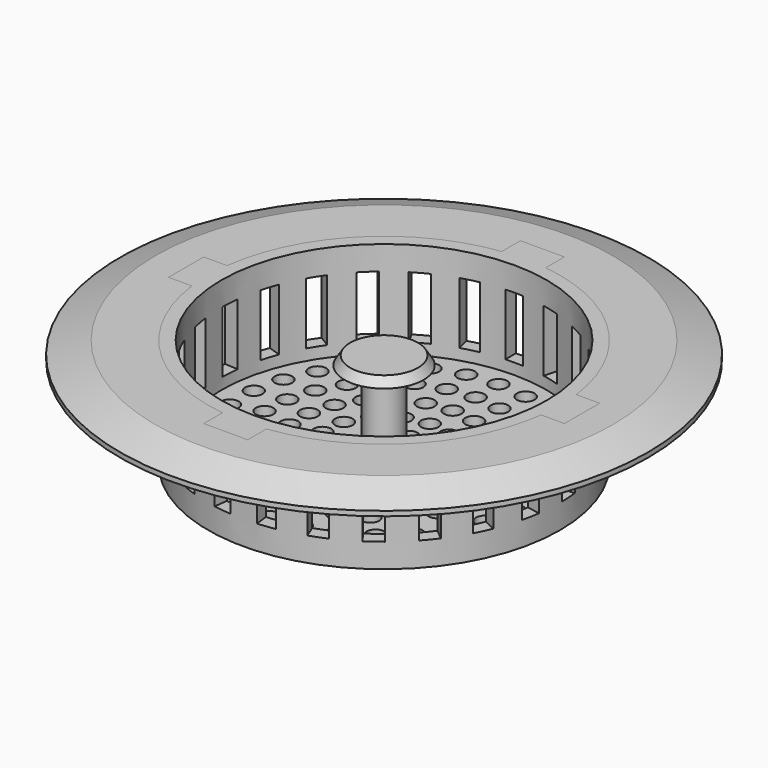
from build123d import *

# Parameters (mm, degrees)
F0_R      = 40
F1_DEPTH  = 25
F2_T      = -3
F4_DEPTH  = 2
F5_R      = 60
F5_R_2    = 40
F6_DEPTH  = 4
F7_DEPTH  = 2
F8_R      = 2
F9_DEPTH  = 3.001
F12_SIZE2 = 2.9117618741
F12_SIZE  = 8
F14_W     = 4
F14_H     = 6.67
F15_DEPTH = 7


# Not quite as in the source:
# - a feature names something its author has since deleted; it is built from what else it names


with BuildPart() as f1:
    # F0 (on Top) → F1 (new body)
    with BuildSketch(Plane.XY):
        Circle(F0_R)
    extrude(amount=F1_DEPTH)

    # F2
    f2_openings = [f1.faces().sort_by_distance(p)[0] for p in [
        (0, 0, 25),
    ]]
    offset(amount=F2_T, openings=f2_openings)

    # F3 (on face) → F4 (join)
    with BuildSketch(Plane.XY.offset(25)):
        with BuildLine():
            ThreePointArc((-39.686269666, -5), (-40, 0), (-39.686269666, 5))
            Line((-39.686269666, 5), (-45, 5))
            Line((-45, 5), (-45, 0))
            Line((-45, 0), (-45, -5))
            Line((-45, -5), (-39.686269666, -5))
        make_face()
        with BuildLine():
            Line((-5, 45), (-5, 39.686269666))
            ThreePointArc((-5, 39.686269666), (0, 40), (5, 39.686269666))
            Line((5, 39.686269666), (5, 45))
            Line((5, 45), (0, 45))
            Line((0, 45), (-5, 45))
        make_face()
        with BuildLine():
            Line((45, 5), (39.686269666, 5))
            ThreePointArc((39.686269666, 5), (39.9214903695, 2.5049165017), (40, 0))
            ThreePointArc((40, 0), (39.9214903695, -2.5049165017), (39.686269666, -5))
            Line((39.686269666, -5), (45, -5))
            Line((45, -5), (45, 0))
            Line((45, 0), (45, 5))
        make_face()
        with BuildLine():
            ThreePointArc((5, -39.686269666), (0, -40), (-5, -39.686269666))
            Line((-5, -39.686269666), (-5, -45))
            Line((-5, -45), (0, -45))
            Line((0, -45), (5, -45))
            Line((5, -45), (5, -39.686269666))
        make_face()
    extrude(amount=-F4_DEPTH)

    # F8 (on face) → F9 (cut, through all)
    with BuildSketch(Plane.XY.offset(3)):
        with Locations((30.9093367796, -10.0430523172)):
            Circle(F8_R)
        with Locations((-19.1030206995, 26.2930523172)):
            Circle(F8_R)
        with Locations((-14.2872334298, -21.7226830967)):
            Circle(F8_R)
        with Locations((-24.9077273202, -7.4568840505)):
            Circle(F8_R)
        with Locations((32.3219615995, -3.3971750562)):
            Circle(F8_R)
        with Locations((-5.4728203773, 4.364428613)):
            Circle(F8_R)
        with Locations((0, 7)):
            Circle(F8_R)
        with Locations((28.145825623, -16.25)):
            Circle(F8_R)
        with Locations((-5.9960126393, 25.2991666351)):
            Circle(F8_R)
        with Locations((32.3219615995, 3.3971750562)):
            Circle(F8_R)
        with Locations((-2.7028519806, -12.7159188095)):
            Circle(F8_R)
        with Locations((16.7124778519, 19.9171555211)):
            Circle(F8_R)
        with Locations((10.5424959404, 16.4044438902)):
            Circle(F8_R)
        with Locations((14.7371166999, 12.7697843119)):
            Circle(F8_R)
        with Locations((30.9093367796, 10.0430523172)):
            Circle(F8_R)
        with Locations((-6.7571299516, -31.7897970238)):
            Circle(F8_R)
        with Locations((-13.2189409, 29.6902273734)):
            Circle(F8_R)
        with Locations((-11.6687786852, 23.2344486484)):
            Circle(F8_R)
        with Locations((19.3015181167, -2.7751393463)):
            Circle(F8_R)
        with Locations((11.6687786852, 23.2344486484)):
            Circle(F8_R)
        with Locations((23.8736187789, 10.298073917)):
            Circle(F8_R)
        with Locations((-23.8736187789, 10.298073917)):
            Circle(F8_R)
        with Locations((-12.3637347118, 4.0172209269)):
            Circle(F8_R)
        with Locations((-30.9093367796, 10.0430523172)):
            Circle(F8_R)
        with Locations((-5.28757636, 11.8760909494)):
            Circle(F8_R)
        with Locations((-11.2583302492, -6.5)):
            Circle(F8_R)
        with Locations((-16.7124778519, 19.9171555211)):
            Circle(F8_R)
        with Locations((-30.9093367796, -10.0430523172)):
            Circle(F8_R)
        with Locations((0, -32.5)):
            Circle(F8_R)
        with Locations((-22.5166604984, -13)):
            Circle(F8_R)
        with Locations((-28.145825623, 16.25)):
            Circle(F8_R)
        with Locations((-14.7371166999, 12.7697843119)):
            Circle(F8_R)
        with Locations((0, 19.5)):
            Circle(F8_R)
        with Locations((0, 26)):
            Circle(F8_R)
        with Locations((7.6412082798, -10.5172209269)):
            Circle(F8_R)
        with Locations((-8.8925237265, -24.4320081404)):
            Circle(F8_R)
        with Locations((-32.3219615995, 3.3971750562)):
            Circle(F8_R)
        with Locations((-19.1030206995, -26.2930523172)):
            Circle(F8_R)
        with Locations((12.3637347118, 4.0172209269)):
            Circle(F8_R)
        with Locations((-3.0184157673, -25.8241973013)):
            Circle(F8_R)
        with Locations((3.0371861738, -6.3067820753)):
            Circle(F8_R)
        with Locations((14.2872334298, -21.7226830967)):
            Circle(F8_R)
        with Locations((-20.8552030116, 15.5261233843)):
            Circle(F8_R)
        with Locations((-25.9560121151, -1.5117655517)):
            Circle(F8_R)
        with Locations((-19.3015181167, -2.7751393463)):
            Circle(F8_R)
        with Locations((24.152206828, -21.7467447067)):
            Circle(F8_R)
        with Locations((8.8925237265, -24.4320081404)):
            Circle(F8_R)
        with Locations((11.2583302492, -6.5)):
            Circle(F8_R)
        with Locations((-6.7571299516, 31.7897970238)):
            Circle(F8_R)
        with Locations((6.7571299516, 31.7897970238)):
            Circle(F8_R)
        with Locations((12.9287846398, -1.3588700225)):
            Circle(F8_R)
        with Locations((5.4937848584, 18.7101129855)):
            Circle(F8_R)
        with Locations((3.0184157673, -25.8241973013)):
            Circle(F8_R)
        with Locations((25.9560121151, -1.5117655517)):
            Circle(F8_R)
        with Locations((-18.9117146809, -17.8422825846)):
            Circle(F8_R)
        with Locations((28.145825623, 16.25)):
            Circle(F8_R)
        with Locations((-7.6412082798, -10.5172209269)):
            Circle(F8_R)
        with Locations((-6.8244953853, -1.5576465377)):
            Circle(F8_R)
        with Locations((25.6050015783, 4.5148526193)):
            Circle(F8_R)
        with Locations((0, 32.5)):
            Circle(F8_R)
        with Locations((-32.3219615995, -3.3971750562)):
            Circle(F8_R)
        with Locations((-10.5424959404, 16.4044438902)):
            Circle(F8_R)
        with Locations((24.152206828, 21.7467447067)):
            Circle(F8_R)
        with Locations((-25.6050015783, 4.5148526193)):
            Circle(F8_R)
        with Locations((5.28757636, 11.8760909494)):
            Circle(F8_R)
        with Locations((13.2189409, 29.6902273734)):
            Circle(F8_R)
        with Locations((19.1030206995, 26.2930523172)):
            Circle(F8_R)
        with Locations((-9.6608827312, 8.6986978827)):
            Circle(F8_R)
        with Locations((-19.3015181167, 2.7751393463)):
            Circle(F8_R)
        with Locations((-10.5424959404, -16.4044438902)):
            Circle(F8_R)
        with Locations((-24.152206828, -21.7467447067)):
            Circle(F8_R)
        with Locations((5.4728203773, 4.364428613)):
            Circle(F8_R)
        with Locations((9.6608827312, 8.6986978827)):
            Circle(F8_R)
        with Locations((0, 13)):
            Circle(F8_R)
        with Locations((19.1030206995, -26.2930523172)):
            Circle(F8_R)
        with Locations((13.2189409, -29.6902273734)):
            Circle(F8_R)
        with Locations((6.7571299516, -31.7897970238)):
            Circle(F8_R)
        with Locations((22.5166604984, -13)):
            Circle(F8_R)
        with Locations((24.9077273202, -7.4568840505)):
            Circle(F8_R)
        with Locations((18.9117146809, -17.8422825846)):
            Circle(F8_R)
        with Locations((-17.7378239094, -8.1005927535)):
            Circle(F8_R)
        with Locations((-17.7378239094, 8.1005927535)):
            Circle(F8_R)
        with Locations((-14.7371166999, -12.7697843119)):
            Circle(F8_R)
        with Locations((10.5424959404, -16.4044438902)):
            Circle(F8_R)
        with Locations((14.7371166999, -12.7697843119)):
            Circle(F8_R)
        with Locations((17.7378239094, 8.1005927535)):
            Circle(F8_R)
        with Locations((20.8552030116, 15.5261233843)):
            Circle(F8_R)
        with Locations((5.9960126393, 25.2991666351)):
            Circle(F8_R)
        with Locations((-5.4937848584, 18.7101129855)):
            Circle(F8_R)
        with Locations((-28.145825623, -16.25)):
            Circle(F8_R)
        with Locations((-24.152206828, 21.7467447067)):
            Circle(F8_R)
        with Locations((0, -19.5)):
            Circle(F8_R)
        with Locations((5.4937848584, -18.7101129855)):
            Circle(F8_R)
        with Locations((-12.9287846398, -1.3588700225)):
            Circle(F8_R)
        with Locations((6.8244953853, -1.5576465377)):
            Circle(F8_R)
        with Locations((-13.2189409, -29.6902273734)):
            Circle(F8_R)
        with Locations((17.7378239094, -8.1005927535)):
            Circle(F8_R)
        with Locations((2.7028519806, -12.7159188095)):
            Circle(F8_R)
        with Locations((-5.4937848584, -18.7101129855)):
            Circle(F8_R)
        with Locations((19.3015181167, 2.7751393463)):
            Circle(F8_R)
        with Locations((-3.0371861738, -6.3067820753)):
            Circle(F8_R)
    extrude(amount=-F9_DEPTH, mode=Mode.SUBTRACT)

    # F10 (on Front) → F11 (revolve)
    with BuildSketch(Plane.XZ):
        Polygon((0, 22), (0, 0), (4, 0), (4, 20), (9, 20), (7.7110708915, 22), align=None)
    revolve(axis=Axis((0, 0, 12.5114747789), (0, 0, -1)))

    # F14 (on offset) → F15 (cut, symmetric)
    with BuildSketch(Plane.XY.offset(12.5)):
        Polygon((-6.4256858452, -34.9070814551), (-7.2616585131, -41.5244865129), (-3.2931997078, -42.0258194471), (-2.45722704, -35.4084143894), align=None)
        with Locations((0, 38.7721806765)):
            Rectangle(F14_W, F14_H)
        Polygon((-15.3193786306, 32.0173454969), (-18.5326756369, 37.8623110528), (-22.037902357, 35.9352963564), (-18.8246053508, 30.0903308005), align=None)
        Polygon((11.1857433132, -33.6849064245), (13.6411340796, -39.8865155854), (17.3602400231, -38.4140173747), (14.9048492567, -32.2124082138), align=None)
        Polygon((-22.8004822195, 27.2016871693), (-27.366411416, 32.0639079142), (-30.2822859257, 29.3257194904), (-25.7163567292, 24.4634987455), align=None)
        Polygon((19.2114181957, -29.8448519046), (23.1319458285, -35.2409952571), (26.368013806, -32.8898542479), (22.4474861732, -27.4937108954), align=None)
        Polygon((26.0299690184, -24.1295355778), (31.1692923477, -28.3811535894), (33.7189883067, -25.2991006183), (28.5796649773, -21.0474826067), align=None)
        Polygon((18.8246053508, 30.0903308005), (22.037902357, 35.9352963564), (18.5326756369, 37.8623110528), (15.3193786306, 32.0173454969), align=None)
        Polygon((2.45722704, -35.4084143894), (3.2931997078, -42.0258194471), (7.2616585131, -41.5244865129), (6.4256858452, -34.9070814551), align=None)
        Polygon((30.9922548362, 17.299535094), (36.6239220993, 20.8734998165), (34.4806149193, 24.2508115185), (28.8489476562, 20.676846796), align=None)
        Polygon((-28.8489476562, 20.676846796), (-34.4806149193, 24.2508115185), (-36.6239220993, 20.8734998165), (-30.9922548362, 17.299535094), align=None)
        Polygon((-35.2416724562, 4.2211724422), (-41.8985107348, 4.6399852074), (-42.1496728129, 0.6478782937), (-35.4928345343, 0.2290655285), align=None)
        Polygon((10.7500347861, 33.8264767068), (12.4087963335, 40.2869263915), (8.534463689, 41.2816859402), (6.8757021416, 34.8212362554), align=None)
        Polygon((-22.4474861732, -27.4937108954), (-26.368013806, -32.8898542479), (-23.1319458285, -35.2409952571), (-19.2114181957, -29.8448519046), align=None)
        Polygon((-14.9048492567, -32.2124082138), (-17.3602400231, -38.4140173747), (-13.6411340796, -39.8865155854), (-11.1857433132, -33.6849064245), align=None)
        Polygon((-6.8757021416, 34.8212362554), (-8.534463689, 41.2816859401), (-12.4087963335, 40.2869263915), (-10.7500347861, 33.8264767068), align=None)
        Polygon((-33.0847276127, 12.8528040944), (-39.4282745764, 14.9139474468), (-40.6643425539, 11.1097213817), (-34.3207955902, 9.0485780292), align=None)
        Polygon((25.7163567292, 24.4634987455), (30.2822859257, 29.3257194904), (27.366411416, 32.0639079142), (22.8004822195, 27.2016871693), align=None)
        Polygon((35.4928345343, 0.2290655285), (42.1496728129, 0.6478782937), (41.8985107348, 4.6399852074), (35.2416724562, 4.2211724422), align=None)
        Polygon((-32.9160783223, -13.2787635786), (-38.9512747623, -16.1187114533), (-37.248157596, -19.7380196632), (-31.2129611561, -16.8980717884), align=None)
        Polygon((-35.1842534094, -4.6756909989), (-41.7361093718, -5.9255243672), (-40.9865841134, -9.8546733701), (-34.4347281511, -8.6048400018), align=None)
        Polygon((-28.5796649773, -21.0474826067), (-33.7189883067, -25.2991006183), (-31.1692923477, -28.3811535894), (-26.0299690184, -24.1295355778), align=None)
        Polygon((34.3207955902, 9.0485780292), (40.6643425539, 11.1097213817), (39.4282745764, 14.9139474468), (33.0847276127, 12.8528040944), align=None)
        Polygon((34.4347281511, -8.6048400018), (40.9865841134, -9.8546733701), (41.7361093718, -5.9255243672), (35.1842534094, -4.6756909989), align=None)
        Polygon((31.2129611561, -16.8980717884), (37.248157596, -19.7380196632), (38.9512747623, -16.1187114533), (32.9160783223, -13.2787635786), align=None)
    extrude(amount=F15_DEPTH, both=True, mode=Mode.SUBTRACT)


with BuildPart() as f6:
    # F5 (on face) → F6 (new body)
    with BuildSketch(Plane.XY.offset(25)):
        Circle(F5_R)
        Circle(F5_R_2, mode=Mode.SUBTRACT)
    extrude(amount=-F6_DEPTH)

    # F3 (on face) → F7 (cut)
    with BuildSketch(Plane.XY.offset(25)):
        with BuildLine():
            Line((-5, 45), (-5, 39.686269666))
            ThreePointArc((-5, 39.686269666), (0, 40), (5, 39.686269666))
            Line((5, 39.686269666), (5, 45))
            Line((5, 45), (0, 45))
            Line((0, 45), (-5, 45))
        make_face()
        with BuildLine():
            Line((45, 5), (39.686269666, 5))
            ThreePointArc((39.686269666, 5), (39.9214903695, 2.5049165017), (40, 0))
            ThreePointArc((40, 0), (39.9214903695, -2.5049165017), (39.686269666, -5))
            Line((39.686269666, -5), (45, -5))
            Line((45, -5), (45, 0))
            Line((45, 0), (45, 5))
        make_face()
        with BuildLine():
            ThreePointArc((5, -39.686269666), (0, -40), (-5, -39.686269666))
            Line((-5, -39.686269666), (-5, -45))
            Line((-5, -45), (0, -45))
            Line((0, -45), (5, -45))
            Line((5, -45), (5, -39.686269666))
        make_face()
        with BuildLine():
            ThreePointArc((-39.686269666, -5), (-40, 0), (-39.686269666, 5))
            Line((-39.686269666, 5), (-45, 5))
            Line((-45, 5), (-45, 0))
            Line((-45, 0), (-45, -5))
            Line((-45, -5), (-39.686269666, -5))
        make_face()
    extrude(amount=-F7_DEPTH, mode=Mode.SUBTRACT)

    # F12
    f12_edges = [f6.edges().sort_by_distance(p)[0] for p in [
        (-60, 0, 25),
    ]]
    f12_side = f6.faces().sort_by_distance((-58.302944, 0, 25))[0]
    chamfer(f12_edges, length=F12_SIZE, length2=F12_SIZE2, reference=f12_side)


solid = Compound([f1.part, f6.part])
